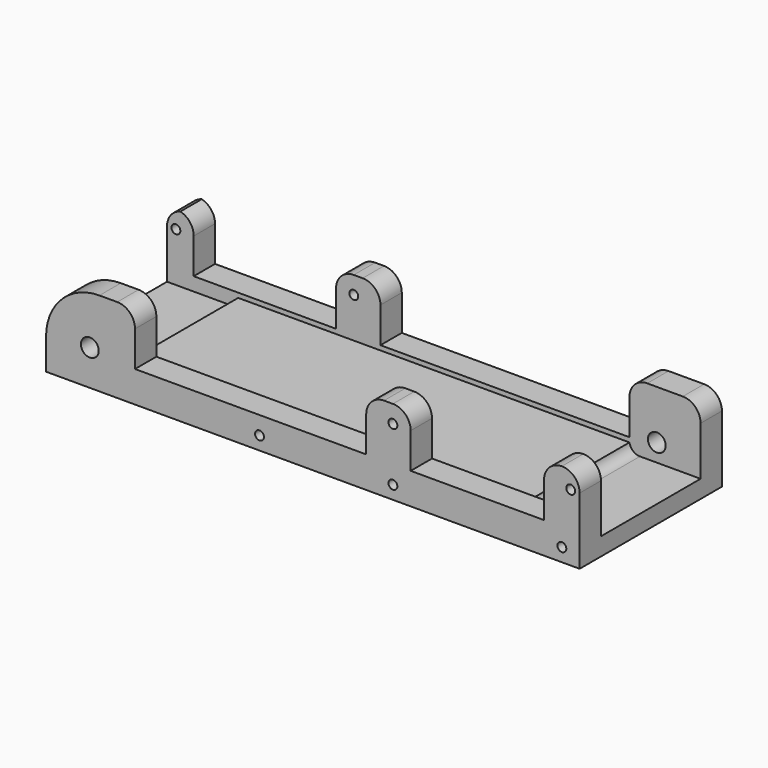
from build123d import *

# Parameters (mm, degrees)
F0_W         = 381
F0_H         = 127
F1_DEPTH     = 60.325
F2_W         = 88.9
F2_H         = 41.275
F3_DEPTH     = 381
F4_W         = 88.9
F4_H         = 6.35
F5_DEPTH     = 50.8
F6_T1_DEPTH  = 126.4671066227
F7_W         = 88.9
F7_H         = 6.35
F8_DEPTH     = 50.8
F9_T1_DEPTH  = 126.4671066227
F10_W        = 165.1
F10_H        = 37.973
F10_W_2      = 95.25
F11_DEPTH    = 19.05
F12_W        = 177.8
F12_H        = 37.973
F12_W_2      = 101.6
F13_DEPTH    = 19.05
F14_R        = 38.1
F15_R        = 12.69999
F16_T1_DEPTH = 82.55
F18_D        = 6.35
F18_DEPTH    = 12.7
F18_TIP      = 1.9077324654
F19_D        = 6.35
F19_DEPTH    = 25.4
F19_TIP      = 1.9077324654
F20_D        = 12.7
F20_DEPTH    = 25.4
F20_TIP      = 3.8154649308
F22_D        = 12.7
F22_DEPTH    = 25.4
F22_TIP      = 3.8154649308
F23_D        = 6.35
F23_DEPTH    = 12.7
F23_TIP      = 1.9077324654
F24_D        = 6.35
F24_DEPTH    = 25.4
F24_TIP      = 1.9077324654


# Not quite as in the source:
# - a fillet or chamfer that OpenCascade refuses, or shapes differently, is made with other operations: its cross-section is extruded or revolved along the edge and cut away or added
# - a fillet or chamfer is up to 0.001 mm smaller than in the source, because OpenCascade refuses the exact size


with BuildPart() as f1:
    # F0 (on Top) → F1 (new body)
    with BuildSketch(Plane.XY):
        Rectangle(F0_W, F0_H)
    extrude(amount=F1_DEPTH)

    # F2 (on face) → F3 (cut, through all)
    with BuildSketch(Plane.YZ.offset(190.5)):
        with Locations((0, 39.6875)):
            Rectangle(F2_W, F2_H)
    extrude(amount=-F3_DEPTH, mode=Mode.SUBTRACT)

    # F4 (on face) → F5 (cut)
    with BuildSketch(Plane.YZ.offset(190.5)):
        with Locations((0, 15.875)):
            Rectangle(F4_W, F4_H)
    extrude(amount=-F5_DEPTH, mode=Mode.SUBTRACT)

    # F6: fillet of radius 7.62 on 1 edges, made by hand

    # F6_s2 → F6_t1 (join)
    with BuildSketch(Plane.XZ.offset(-63.2335533113)):
        with BuildLine():
            ThreePointArc((139.7, 19.05), (142.2947324749, 14.5001288674), (147.2134213245, 12.7))
            Line((147.2134213245, 12.7), (139.7, 12.7))
            Line((139.7, 12.7), (139.7, 19.05))
        make_face()
    extrude(amount=F6_T1_DEPTH)

    # F7 (on face) → F8 (cut)
    with BuildSketch(Plane(origin=(-190.5, 0, 0), x_dir=(0, -1, 0), z_dir=(-1, 0, 0))):
        with Locations((0, 15.875)):
            Rectangle(F7_W, F7_H)
    extrude(amount=-F8_DEPTH, mode=Mode.SUBTRACT)

    # F9: fillet of radius 7.62 on 1 edges, made by hand

    # F9_s2 → F9_t1 (join)
    with BuildSketch(Plane.XZ.offset(-63.2335533113)):
        with BuildLine():
            ThreePointArc((-147.2134213245, 12.7), (-142.2947324749, 14.5001288674), (-139.7, 19.05))
            Line((-139.7, 19.05), (-139.7, 12.7))
            Line((-139.7, 12.7), (-147.2134213245, 12.7))
        make_face()
    extrude(amount=F9_T1_DEPTH)

    # F10 (on face) → F11 (cut, through all)
    with BuildSketch(Plane.XZ.offset(63.5)):
        with Locations((-44.45, 41.3385)):
            Rectangle(F10_W, F10_H)
        with Locations((117.475, 41.3385)):
            Rectangle(F10_W_2, F10_H)
    extrude(amount=-F11_DEPTH, mode=Mode.SUBTRACT)

    # F12 (on face) → F13 (cut, through all)
    with BuildSketch(Plane(origin=(0, 63.5, 0), x_dir=(-1, 0, 0), z_dir=(0, 1, 0))):
        with Locations((-50.8, 41.3385)):
            Rectangle(F12_W, F12_H)
        with Locations((120.65, 41.3385)):
            Rectangle(F12_W_2, F12_H)
    extrude(amount=-F13_DEPTH, mode=Mode.SUBTRACT)

    # F14
    f14_edges = [f1.edges().sort_by_distance(p)[0] for p in [
        (-190.5, -53.975, 60.325),
    ]]
    fillet(f14_edges, radius=F14_R)

    # F15 (radius 12.7 in the source; OpenCascade refuses exactly that, so slightly less here)
    f15_edges = [f1.edges().sort_by_distance(p)[0] for p in [
        (-127, -53.975, 60.325),
        (38.1, -53.975, 60.325),
        (69.85, -53.975, 60.325),
        (165.1, -53.975, 60.325),
        (190.5, -53.975, 60.325),
    ]]
    fillet(f15_edges, radius=F15_R)

    # F16: fillet of radius 12.7 on 6 edges, made by hand

    # F16_s2 → F16_t1 (cut)
    with BuildSketch(Plane.XZ.offset(-95.25)):
        with BuildLine():
            ThreePointArc((-184.15, 60.325), (-175.1697438789, 56.6052561211), (-171.45, 47.625))
            Line((-171.45, 47.625), (-171.45, 60.325))
            Line((-171.45, 60.325), (-184.15, 60.325))
        make_face()
        with BuildLine():
            ThreePointArc((-190.5, 47.625), (-186.7802561211, 56.6052561211), (-177.8, 60.325))
            Line((-177.8, 60.325), (-190.5, 60.325))
            Line((-190.5, 60.325), (-190.5, 47.625))
        make_face()
        with BuildLine():
            ThreePointArc((-57.15, 60.325), (-66.1302561211, 56.6052561211), (-69.85, 47.625))
            Line((-69.85, 47.625), (-69.85, 60.325))
            Line((-69.85, 60.325), (-57.15, 60.325))
        make_face()
        with BuildLine():
            ThreePointArc((-38.1, 47.625), (-41.8197438789, 56.6052561211), (-50.8, 60.325))
            Line((-50.8, 60.325), (-38.1, 60.325))
            Line((-38.1, 60.325), (-38.1, 47.625))
        make_face()
        with BuildLine():
            ThreePointArc((152.4, 60.325), (143.4197438789, 56.6052561211), (139.7, 47.625))
            Line((139.7, 47.625), (139.7, 60.325))
            Line((139.7, 60.325), (152.4, 60.325))
        make_face()
        with BuildLine():
            ThreePointArc((190.5, 47.625), (186.7802561211, 56.6052561211), (177.8, 60.325))
            Line((177.8, 60.325), (190.5, 60.325))
            Line((190.5, 60.325), (190.5, 47.625))
        make_face()
    extrude(amount=F16_T1_DEPTH, mode=Mode.SUBTRACT)

    # F18
    with Locations(Plane.XZ.offset(63.5)):
        with Locations((-38.1, 9.525), (57.15, 9.525), (177.8, 9.525)):
            Hole(F18_D / 2, depth=F18_DEPTH)
            with Locations((0, 0, -(F18_DEPTH + F18_TIP / 2))):  # 118° drill point
                Cone(0, F18_D / 2, F18_TIP, mode=Mode.SUBTRACT)

    # F19
    with Locations(Plane.XZ.offset(63.5)):
        with Locations((57.15, 47.752), (184.15, 47.752)):
            Hole(F19_D / 2, depth=F19_DEPTH)
            with Locations((0, 0, -(F19_DEPTH + F19_TIP / 2))):  # 118° drill point
                Cone(0, F19_D / 2, F19_TIP, mode=Mode.SUBTRACT)

    # F20
    with Locations(Plane.XZ.offset(63.5)):
        with Locations((-159.258, 25.4)):
            Hole(F20_D / 2, depth=F20_DEPTH)
            with Locations((0, 0, -(F20_DEPTH + F20_TIP / 2))):  # 118° drill point
                Cone(0, F20_D / 2, F20_TIP, mode=Mode.SUBTRACT)

    # F22
    with Locations(Plane(origin=(0, 63.5, 0), x_dir=(-1, 0, 0), z_dir=(0, 1, 0))):
        with Locations((-159.258, 25.4)):
            Hole(F22_D / 2, depth=F22_DEPTH)
            with Locations((0, 0, -(F22_DEPTH + F22_TIP / 2))):  # 118° drill point
                Cone(0, F22_D / 2, F22_TIP, mode=Mode.SUBTRACT)

    # F23
    with Locations(Plane(origin=(0, 63.5, 0), x_dir=(-1, 0, 0), z_dir=(0, 1, 0))):
        with Locations((-38.1, 9.652), (57.15, 9.652), (177.8, 9.652)):
            Hole(F23_D / 2, depth=F23_DEPTH)
            with Locations((0, 0, -(F23_DEPTH + F23_TIP / 2))):  # 118° drill point
                Cone(0, F23_D / 2, F23_TIP, mode=Mode.SUBTRACT)

    # F24
    with Locations(Plane(origin=(0, 63.5, 0), x_dir=(-1, 0, 0), z_dir=(0, 1, 0))):
        with Locations((57.15, 47.752), (184.15, 47.752)):
            Hole(F24_D / 2, depth=F24_DEPTH)
            with Locations((0, 0, -(F24_DEPTH + F24_TIP / 2))):  # 118° drill point
                Cone(0, F24_D / 2, F24_TIP, mode=Mode.SUBTRACT)


solid = f1.part
